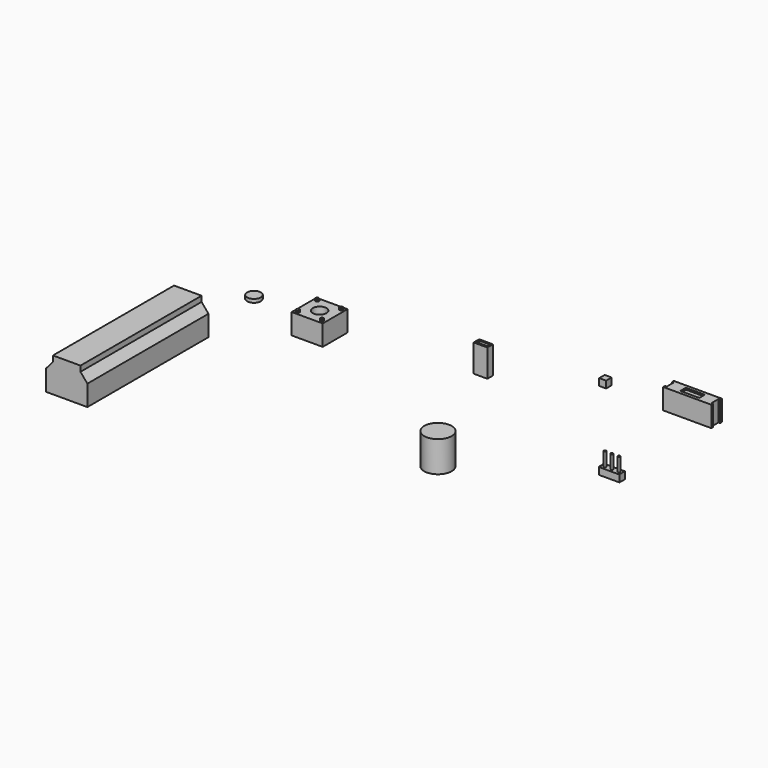
from build123d import *

# Parameters (mm, degrees)
F0_R      = 3.175
F1_DEPTH  = 7.14375
F3_DEPTH  = 34.925
F4_W      = 7.14375
F4_H      = 7.14375
F4_R      = 0.396875
F4_R_2    = 1.5875
F5_DEPTH  = 4.7625
F6_DEPTH  = 5.159375
F8_DEPTH  = 4.7625
F9_W      = 4.365625
F9_H      = 1.6002
F10_DEPTH = 0.396875
F11_W     = 1.5875
F11_H     = 1.5875
F12_DEPTH = 1.6002
F13_W     = 4.7625
F13_H     = 1.6002
F13_R     = 0.2645833333
F14_DEPTH = 1.6002
F15_DEPTH = 4.7625
F16_W     = 3.175
F16_H     = 1.6002
F17_DEPTH = 6.35
F18_W     = 2.38125
F18_H     = 0.80645
F19_DEPTH = 6.096
F20_W     = 0.0608872609
F20_H     = 1.6002
F20_W_2   = 0.0508
F21_DEPTH = 0.0508
F22_R     = 1.5875
F23_DEPTH = 0.79375


# Not quite as in the source:
# - a length typed as a fraction of an inch, garbled in the dataset ("3 / 203.2 mm" for 3/8 in), is restored


with BuildPart() as f1:
    # F0 (on Top) → F1 (new body)
    with BuildSketch(Plane.XY):
        Circle(F0_R)
    extrude(amount=F1_DEPTH)


with BuildPart() as f3:
    # F2 (on Front) → F3 (new body)
    with BuildSketch(Plane.XZ):
        Polygon((-60.8911556599, 15.6311627035), (-62.4786556599, 13.7401700254), (-62.4786556599, 8.9776700254), (-52.9536556599, 8.9776700254), (-52.9536556599, 13.7401700254), (-54.5411556599, 15.6311627035), (-54.5411556599, 16.8918247443), (-60.8911556599, 16.8918247443), align=None)
    extrude(amount=F3_DEPTH)


with BuildPart() as f5:
    # F4 (on Top) → F5 (new body)
    with BuildSketch(Plane.XY):
        with Locations((-48.8571682945, 26.9388640299)):
            Rectangle(F4_W, F4_H)
        with Locations((-51.6352932945, 24.1607390299)):
            Circle(F4_R, mode=Mode.SUBTRACT)
        with Locations((-46.0790432945, 24.1607390299)):
            Circle(F4_R, mode=Mode.SUBTRACT)
        with Locations((-51.6352932945, 29.7169890299)):
            Circle(F4_R, mode=Mode.SUBTRACT)
        with Locations((-48.8571682945, 26.9388640299)):
            Circle(F4_R_2, mode=Mode.SUBTRACT)
        with Locations((-46.0790432945, 29.7169890299)):
            Circle(F4_R, mode=Mode.SUBTRACT)
    extrude(amount=F5_DEPTH)

    # F4 (on Top) → F6 (join)
    with BuildSketch(Plane.XY):
        with Locations((-51.6352932945, 29.7169890299)):
            Circle(F4_R)
        with Locations((-46.0790432945, 29.7169890299)):
            Circle(F4_R)
        with Locations((-46.0790432945, 24.1607390299)):
            Circle(F4_R)
        with Locations((-51.6352932945, 24.1607390299)):
            Circle(F4_R)
    extrude(amount=F6_DEPTH)


with BuildPart() as f8:
    # F7 (on Top) → F8 (new body)
    with BuildSketch(Plane.XY):
        Polygon((29.2134701102, 45.3868062362), (18.1009701102, 45.3868062362), (18.1009701102, 44.8576395696), (18.4978451102, 44.8576395696), (18.4978451102, 42.8732645696), (18.1009701102, 42.8732645696), (18.1009701102, 42.3440979029), (29.2134701102, 42.3440979029), (29.2134701102, 42.8732645696), (28.8165951102, 42.8732645696), (28.8165951102, 44.8576395696), (29.2134701102, 44.8576395696), align=None)
    extrude(amount=F8_DEPTH)

    # F9 (on face) → F10 (cut)
    with BuildSketch(Plane.XY.offset(4.7625)):
        with Locations((23.6572201102, 43.8654520696)):
            Rectangle(F9_W, F9_H)
    extrude(amount=-F10_DEPTH, mode=Mode.SUBTRACT)


with BuildPart() as f12:
    # F11 (on Top) → F12 (new body)
    with BuildSketch(Plane.XY):
        with Locations((3.9349747822, 43.3876775205)):
            Rectangle(F11_W, F11_H)
    extrude(amount=F12_DEPTH)


with BuildPart() as f14:
    # F13 (on Top) → F14 (new body)
    with BuildSketch(Plane.XY):
        with Locations((27.1214717252, 16.2639711052)):
            Rectangle(F13_W, F13_H)
        with Locations((25.5339717252, 16.2639711052)):
            Circle(F13_R, mode=Mode.SUBTRACT)
        with Locations((27.1341717252, 16.2639711052)):
            Circle(F13_R, mode=Mode.SUBTRACT)
        with Locations((28.7343717252, 16.2639711052)):
            Circle(F13_R, mode=Mode.SUBTRACT)
    extrude(amount=F14_DEPTH)

    # F13 (on Top) → F15 (join)
    with BuildSketch(Plane.XY):
        with Locations((25.5339717252, 16.2639711052)):
            Circle(F13_R)
        with Locations((27.1341717252, 16.2639711052)):
            Circle(F13_R)
        with Locations((28.7343717252, 16.2639711052)):
            Circle(F13_R)
    extrude(amount=F15_DEPTH)

    # F20 (on face) → F21 (join)
    with BuildSketch(Plane.XY.offset(1.6002)):
        with Locations((24.7706653557, 16.2639711052)):
            Rectangle(F20_W, F20_H)
        with Locations((29.4773217252, 16.2639711052)):
            Rectangle(F20_W_2, F20_H)
    extrude(amount=F21_DEPTH)


with BuildPart() as f17:
    # F16 (on Top) → F17 (new body)
    with BuildSketch(Plane.XY):
        with Locations((-15.9334428608, 32.9927906)):
            Rectangle(F16_W, F16_H)
    extrude(amount=F17_DEPTH)

    # F18 (on face) → F19 (cut)
    with BuildSketch(Plane.XY.offset(6.35)):
        with Locations((-15.9334428608, 32.9927906)):
            Rectangle(F18_W, F18_H)
    extrude(amount=-F19_DEPTH, mode=Mode.SUBTRACT)


with BuildPart() as f23:
    # F22 (on Top) → F23 (new body)
    with BuildSketch(Plane.XY):
        with Locations((-66.6881874204, 30.300328508)):
            Circle(F22_R)
    extrude(amount=F23_DEPTH)


solid = Compound([f1.part, f3.part, f5.part, f8.part, f12.part, f14.part, f17.part, f23.part])
